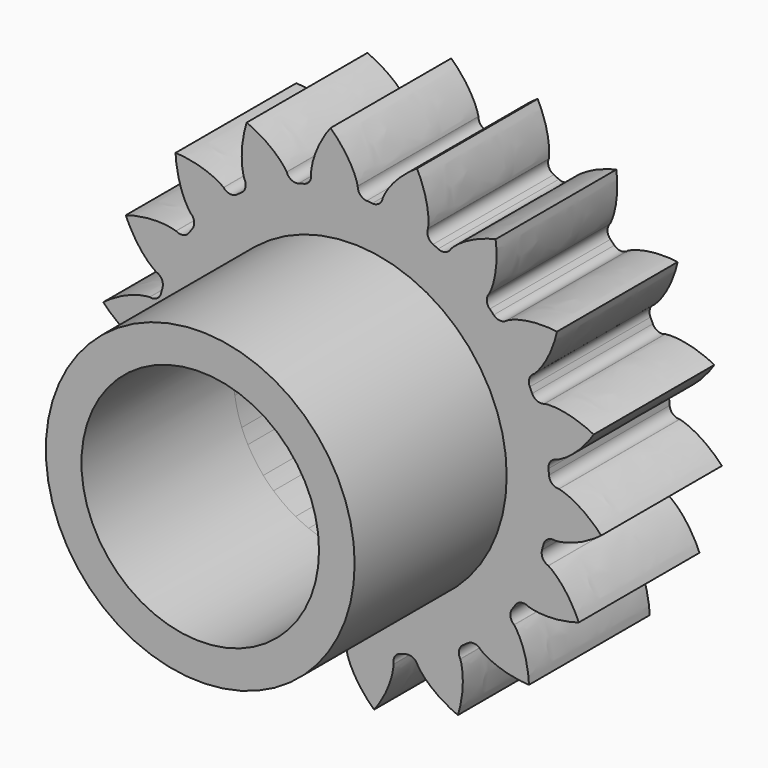
from build123d import *

# Parameters (mm, degrees)
F3_DEPTH        = 3.175
F3_COPIES_COUNT = 18
F4_R            = 0.2032
F6_R            = 3.25
F6_R_2          = 2.499995
F7_DEPTH        = 4


# Not quite as in the source:
# - a feature of the source that left no trace in its solid (it failed there, or was rolled back) is left out
# - a pattern or mirror of a feature is missing from the dataset's text; its kind, count and spacing are read off the source's solid


with BuildPart() as f3:
    # F2 (on Front) → F3 (new body)
    with BuildSketch(Plane.XZ):
        with BuildLine():
            add(Edge.make_bspline(
                [(-0.4583723173, 5.2392195605), (-0.3278673997, 5.109437098), (-0.3658838021, 5.1529612637), (-0.1789892117, 4.938989646), (-0.0876848832, 4.8047332353), (-0.002802043, 4.6596060557), (0.0505409626, 4.5504639736), (0.1012756339, 4.4067213455), (0.0914851093, 4.4344600829), (0.1146747244, 4.3513086339)],
                knots=[0.0115022154, 0.0115022154, 0.0115022154, 0.0115022154, 0.174206303, 0.3392825571, 0.4945901329, 0.6393737619, 0.7727132879, 0.893442598, 1, 1, 1, 1], degree=3))
            add(Edge.make_bspline(
                [(-0.4583723173, 5.2392195605), (-0.5643580838, 5.0887468441), (-0.534477128, 5.1382112589), (-0.6813765882, 4.8950364459), (-0.7479804177, 4.7469648614), (-0.8063726266, 4.5893027393), (-0.8399529083, 4.472555855), (-0.8649561605, 4.3221870171), (-0.8601311573, 4.3512044476), (-0.8685293724, 4.2652894215)],
                knots=[0.0115022154, 0.0115022154, 0.0115022154, 0.0115022154, 0.174206303, 0.3392825571, 0.4945901329, 0.6393737619, 0.7727132879, 0.893442598, 1, 1, 1, 1], degree=3))
            Line((-0.8685293724, 4.2652894215), (-0.8281109962, 4.0667974902))
            ThreePointArc((-0.8281109962, 4.0667974902), (-0.3617184845, 4.1344611966), (0.1093381563, 4.1488136636))
            Line((0.1093381563, 4.1488136636), (0.1146747244, 4.3513086339))
        make_face()
        with BuildLine():
            Line((0.0658621937, 2.499127282), (0.1093381563, 4.1488136636))
            ThreePointArc((0.1093381563, 4.1488136636), (-0.3617184845, 4.1344611966), (-0.8281109962, 4.0667974902))
            Line((-0.8281109962, 4.0667974902), (-0.4988304973, 2.4497230731))
            ThreePointArc((-0.4988304973, 2.4497230731), (-0.2178889211, 2.4904817643), (0.0658621937, 2.499127282))
        make_face()
        with BuildLine():
            ThreePointArc((4.1502541667, 0), (2.9730784371, 2.8957579758), (0.1093381563, 4.1488136636))
            Line((0.1093381563, 4.1488136636), (0.0658621937, 2.499127282))
            ThreePointArc((0.0658621937, 2.499127282), (1.7908978412, 1.7443221957), (2.499995, 0))
            ThreePointArc((2.499995, 0), (-1.5815974916, -1.9361106308), (-0.4988304973, 2.4497230731))
            Line((-0.4988304973, 2.4497230731), (-0.8281109962, 4.0667974902))
            ThreePointArc((-0.8281109962, 4.0667974902), (-2.6256178831, -3.2141469133), (4.1502541667, 0))
        make_face()
    extrude(amount=F3_DEPTH)

    # F3_copies: F3 ×18 about axis
    f3_copies_axis = Axis((0, 0, 0), (0, 1, 0))


with BuildPart() as f3_1:
    add(f3.part)
    for i in range(1, F3_COPIES_COUNT):
        add(f3.part.rotate(f3_copies_axis, i * 360 / F3_COPIES_COUNT))

    # F4
    f4_edges = [f3_1.edges().sort_by_distance(p)[0] for p in [
        (-0.828111, -1.5875, 4.066797),
        (-1.316234, -1.5875, 3.936005),
        (-2.169096, -1.5875, 3.538309),
        (-2.583048, -1.5875, 3.248457),
        (-3.248457, -1.5875, 2.583048),
        (-3.538309, -1.5875, 2.169096),
        (-3.936005, -1.5875, 1.316234),
        (-4.066797, -1.5875, 0.828111),
        (-4.148814, -1.5875, -0.109338),
        (-4.10477, -1.5875, -0.612757),
        (-3.861214, -1.5875, -1.521722),
        (-3.647647, -1.5875, -1.979717),
        (-3.107894, -1.5875, -2.750564),
        (-2.750564, -1.5875, -3.107894),
        (-1.979717, -1.5875, -3.647647),
        (-1.521722, -1.5875, -3.861214),
        (-0.612757, -1.5875, -4.10477),
        (-0.109338, -1.5875, -4.148814),
        (0.828111, -1.5875, -4.066797),
        (1.316234, -1.5875, -3.936005),
        (2.169096, -1.5875, -3.538309),
        (2.583048, -1.5875, -3.248457),
        (3.248457, -1.5875, -2.583048),
        (3.538309, -1.5875, -2.169096),
        (3.936005, -1.5875, -1.316234),
        (4.066797, -1.5875, -0.828111),
        (4.148814, -1.5875, 0.109338),
        (4.10477, -1.5875, 0.612757),
        (3.861214, -1.5875, 1.521722),
        (3.647647, -1.5875, 1.979717),
        (3.107894, -1.5875, 2.750564),
        (2.750564, -1.5875, 3.107894),
        (1.979717, -1.5875, 3.647647),
        (1.521722, -1.5875, 3.861214),
        (0.612757, -1.5875, 4.10477),
        (0.109338, -1.5875, 4.148814),
    ]]
    fillet(f4_edges, radius=F4_R)

    # F6 (on face) → F7 (join)
    with BuildSketch(Plane.XZ.offset(3.175)):
        Circle(F6_R)
        Circle(F6_R_2, mode=Mode.SUBTRACT)
    extrude(amount=F7_DEPTH)


solid = f3_1.part
